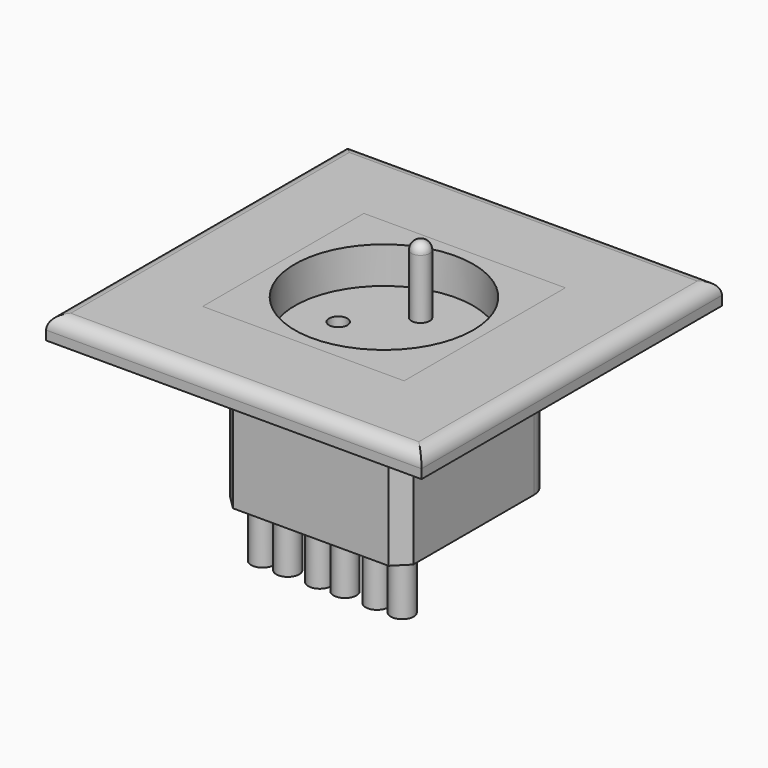
from build123d import *

# Parameters (mm, degrees)
F0_W      = 44
F0_H      = 44
F0_W_2    = 40
F0_H_2    = 40
F0_R      = 19.5
F1_DEPTH  = 8
F0_R_2    = 2
F2_DEPTH  = 30
F3_DEPTH  = 15
F4_R      = 2
F5_W      = 82
F5_H      = 82
F5_W_2    = 44
F5_H_2    = 44
F6_DEPTH  = 5
F9_DEPTH  = 82.001
F10_DEPTH = 82.001
F11_R     = 4
F12_SIZE  = 3
F13_R     = 2.5
F14_DEPTH = 12


with BuildPart() as f1:
    # F0 (on Top) → F1 (new body)
    with BuildSketch(Plane.XY):
        with Locations((0.3887694329, 4.0801210612)):
            Rectangle(F0_W, F0_H)
        with Locations((0.3887694329, 4.0801210612)):
            Rectangle(F0_W_2, F0_H_2, mode=Mode.SUBTRACT)
        with Locations((0.3887694329, 4.0801210612)):
            Rectangle(F0_W_2, F0_H_2)
        with Locations((0.3887694329, 4.0801210612)):
            Circle(F0_R, mode=Mode.SUBTRACT)
    extrude(amount=F1_DEPTH)

    # F0 (on Top) → F2 (join)
    with BuildSketch(Plane.XY):
        with Locations((0.3887694329, 4.0801210612)):
            Rectangle(F0_W_2, F0_H_2)
        with Locations((0.3887694329, 4.0801210612)):
            Circle(F0_R, mode=Mode.SUBTRACT)
        with Locations((0.3887694329, 4.0801210612)):
            Circle(F0_R)
        with Locations((-9.6112305671, 4.0801210612)):
            Circle(F0_R_2, mode=Mode.SUBTRACT)
        with Locations((10.3887694329, 4.0801210612)):
            Circle(F0_R_2, mode=Mode.SUBTRACT)
        with Locations((0.3887694329, 14.0801210612)):
            Circle(F0_R_2, mode=Mode.SUBTRACT)
        with Locations((0.3887694329, 14.0801210612)):
            Circle(F0_R_2)
    extrude(amount=-F2_DEPTH)

    # F0 (on Top) → F3 (join)
    with BuildSketch(Plane.XY):
        with Locations((0.3887694329, 14.0801210612)):
            Circle(F0_R_2)
    extrude(amount=F3_DEPTH)

    # F4
    f4_edges = [f1.edges().sort_by_distance(p)[0] for p in [
        (-1.611231, 14.080121, 15),
    ]]
    fillet(f4_edges, radius=F4_R)

    # F11
    f11_edges = [f1.edges().sort_by_distance(p)[0] for p in [
        (20.388769, 24.080121, -15),
    ]]
    fillet(f11_edges, radius=F11_R)

    # F12
    f12_edges = [f1.edges().sort_by_distance(p)[0] for p in [
        (16.388769, 24.080121, -15),
        (-19.611231, 24.080121, -15),
        (-19.611231, -15.919879, -15),
        (20.388769, -15.919879, -15),
    ]]
    chamfer(f12_edges, length=F12_SIZE)

    # F13 (on face) → F14 (join)
    with BuildSketch(Plane(origin=(0, 0, -30), x_dir=(1, 0, 0), z_dir=(0, 0, -1))):
        with Locations((10.0634490028, 9.9198789388)):
            Circle(F13_R)
        with Locations((3.0634490028, 9.9198789388)):
            Circle(F13_R)
        with Locations((15.5634490028, 9.9198789388)):
            Circle(F13_R)
        with Locations((-2.4365509972, 9.9198789388)):
            Circle(F13_R)
        with Locations((-9.4365509972, 9.9198789388)):
            Circle(F13_R)
        with Locations((-14.9365509972, 9.9198789388)):
            Circle(F13_R)
    extrude(amount=F14_DEPTH)


with BuildPart() as f6:
    # F5 (on face) → F6 (new body)
    with BuildSketch(Plane.XY.offset(8)):
        with Locations((0.3887694329, 4.0801210612)):
            Rectangle(F5_W, F5_H)
        with Locations((0.3887694329, 4.0801210612)):
            Rectangle(F5_W_2, F5_H_2, mode=Mode.SUBTRACT)
    extrude(amount=-F6_DEPTH)

    # F7 (on face) → F9 (cut, through all)
    with BuildSketch(Plane(origin=(-40.6112305671, 0, 0), x_dir=(0, -1, 0), z_dir=(-1, 0, 0))):
        with BuildLine():
            ThreePointArc((-45.0801210612, 5), (-44.2014414048, 7.1213203436), (-42.0801210612, 8))
            Line((-42.0801210612, 8), (-45.0801210612, 8))
            Line((-45.0801210612, 8), (-45.0801210612, 5))
        make_face()
        with BuildLine():
            ThreePointArc((33.9198789388, 8), (36.0411992823, 7.1213203436), (36.9198789388, 5))
            Line((36.9198789388, 5), (36.9198789388, 8))
            Line((36.9198789388, 8), (33.9198789388, 8))
        make_face()
    extrude(amount=-F9_DEPTH, mode=Mode.SUBTRACT)

    # F8 (on face) → F10 (cut, through all)
    with BuildSketch(Plane.XZ.offset(36.9198789388)):
        with BuildLine():
            Line((41.3887694329, 8), (38.3887694329, 8))
            ThreePointArc((38.3887694329, 8), (40.5100897765, 7.1213203436), (41.3887694329, 5))
            Line((41.3887694329, 5), (41.3887694329, 8))
        make_face()
        with BuildLine():
            ThreePointArc((-40.6112305671, 5), (-39.7325509107, 7.1213203436), (-37.6112305671, 8))
            Line((-37.6112305671, 8), (-40.6112305671, 8))
            Line((-40.6112305671, 8), (-40.6112305671, 5))
        make_face()
    extrude(amount=-F10_DEPTH, mode=Mode.SUBTRACT)


solid = Compound([f1.part, f6.part])
